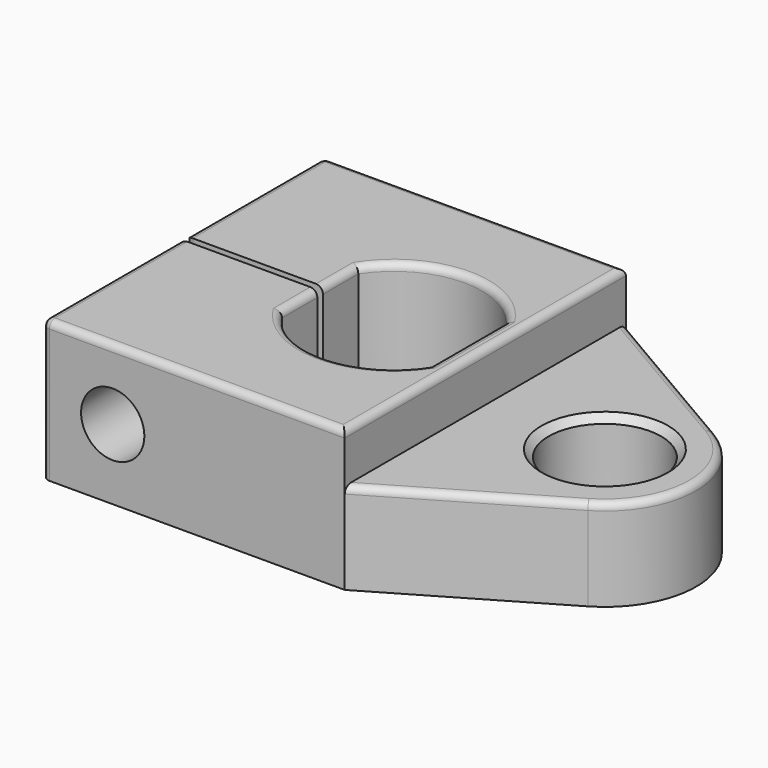
from build123d import *

# Parameters (mm, degrees)
F0_R           = 8
F1_DEPTH       = 13
F2_DEPTH       = 20
F4_D           = 9
F4_CBORE_D     = 15
F4_CBORE_DEPTH = 10
F5_R           = 1
F6_SIZE2       = 1
F6_SIZE        = 1


with BuildPart() as f1:
    # F0 (on Top) → F1 (new body)
    with BuildSketch(Plane.XY):
        with BuildLine():
            Line((43, 50), (43, 0))
            Line((43, 0), (66.5621155816, 13.7777614045))
            ThreePointArc((66.5621155816, 13.7777614045), (73, 25), (66.5621155816, 36.2222385955))
            Line((66.5621155816, 36.2222385955), (43, 50))
        make_face()
        with Locations((60, 25)):
            Circle(F0_R, mode=Mode.SUBTRACT)
    extrude(amount=F1_DEPTH)

    # F0 (on Top) → F2 (join)
    with BuildSketch(Plane.XY):
        with BuildLine():
            Line((0, 24.5), (0, 0))
            Line((0, 0), (43, 0))
            Line((43, 0), (43, 50))
            Line((43, 50), (0, 50))
            Line((0, 50), (0, 25.5))
            Line((0, 25.5), (19.5, 25.5))
            Line((19.5, 25.5), (19.5, 31.7823299831))
            ThreePointArc((19.5, 31.7823299831), (30, 37.5), (40.5, 31.7823299831))
            Line((40.5, 31.7823299831), (40.5, 18.2176700169))
            ThreePointArc((40.5, 18.2176700169), (30, 12.5), (19.5, 18.2176700169))
            Line((19.5, 18.2176700169), (19.5, 24.5))
            Line((19.5, 24.5), (0, 24.5))
        make_face()
    extrude(amount=F2_DEPTH)

    # F4 (through all)
    with Locations(Plane(origin=(0, 50, 0), x_dir=(-1, 0, 0), z_dir=(0, 1, 0))):
        with Locations((-10, 10)):
            CounterBoreHole(F4_D / 2, F4_CBORE_D / 2, F4_CBORE_DEPTH)

    # F5
    f5_edges = [f1.edges().sort_by_distance(p)[0] for p in [
        (0, 0, 10),
        (21.5, 50, 20),
        (0, 37.75, 20),
        (21.5, 0, 20),
        (43, 25, 20),
        (30, 37.5, 20),
        (30, 12.5, 20),
        (40.5, 25, 20),
        (19.5, 21.358835, 20),
        (19.5, 28.641165, 20),
        (0, 25.5, 10),
        (54.781058, 6.888881, 13),
        (0, 12.25, 20),
        (0, 24.5, 10),
        (0, 50, 10),
        (54.781058, 43.111119, 13),
        (73, 25, 13),
    ]]
    fillet(f5_edges, radius=F5_R)

    # F6
    f6_edges = [f1.edges().sort_by_distance(p)[0] for p in [
        (52, 25, 13),
        (17.5, 50, 10),
    ]]
    chamfer(f6_edges, length=F6_SIZE, length2=F6_SIZE2)


solid = f1.part
